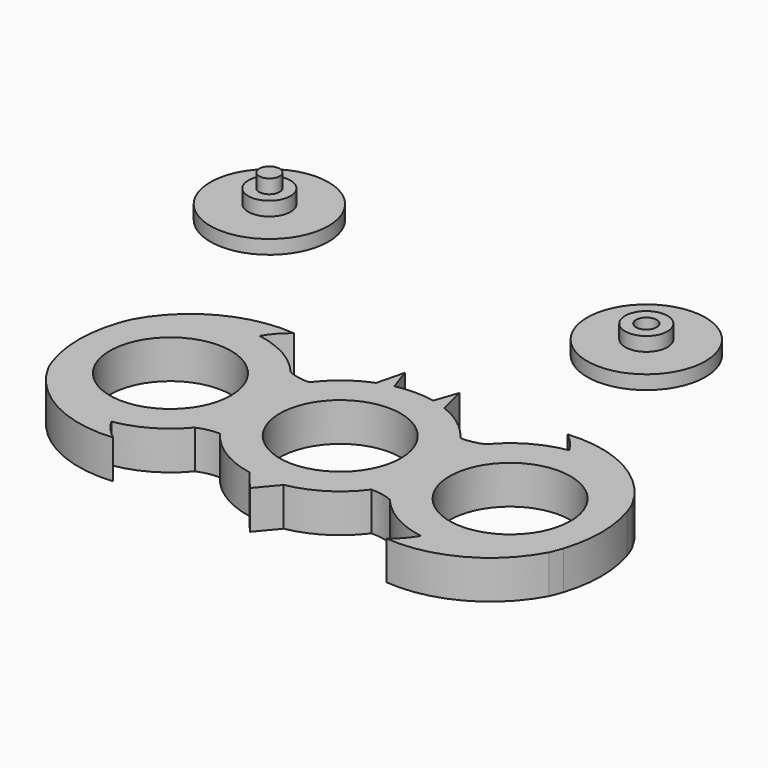
from build123d import *

# Parameters (mm, degrees)
F0_R     = 11.055
F1_DEPTH = 7.04
F2_R     = 3.8608
F2_R_2   = 1.8669
F3_DEPTH = 5.08
F2_R_3   = 10.795
F4_DEPTH = 2.54
F5_DEPTH = 7.62


with BuildPart() as f1:
    # F0 (on Top) → F1 (new body)
    with BuildSketch(Plane.XY):
        with BuildLine():
            ThreePointArc((-46.5429451347, 7.2365655902), (-39.0213444379, 15.1528564439), (-28.2458606842, 16.9223444484))
            ThreePointArc((-28.2458606842, 16.9223444484), (-26.7954522093, 18.9396770038), (-24.9616837395, 20.6161639804))
            ThreePointArc((-24.9616837395, 20.6161639804), (-37.0112899435, 18.1759091976), (-45.6916782608, 9.4696636386))
            ThreePointArc((-45.6916782608, 9.4696636386), (-46.1457401666, 8.3639516727), (-46.5429451347, 7.2365655902))
        make_face()
        with BuildLine():
            ThreePointArc((-28.2458606842, -16.9223444484), (-39.0213444379, -15.1528564439), (-46.5429451347, -7.2365655902))
            ThreePointArc((-46.5429451347, -7.2365655902), (-46.1457401666, -8.3639516727), (-45.6916782608, -9.4696636386))
            ThreePointArc((-45.6916782608, -9.4696636386), (-37.0112899435, -18.1759091976), (-24.9616837395, -20.6161639804))
            ThreePointArc((-24.9616837395, -20.6161639804), (-26.7954522093, -18.9396770038), (-28.2458606842, -16.9223444484))
        make_face()
        with BuildLine():
            ThreePointArc((-13.8011629931, 10.1724591441), (-15.8450830005, 10.3315929693), (-17.8017727644, 10.9433917429))
            ThreePointArc((-17.8017727644, 10.9433917429), (-16.5374743475, 9.2079518218), (-15.5, 7.3280983208))
            ThreePointArc((-15.5, 7.3280983208), (-14.7194475205, 8.7914099944), (-13.8011629931, 10.1724591441))
        make_face()
        with BuildLine():
            ThreePointArc((-13.855, 0), (-14.27130422, 3.7552313511), (-15.5, 7.3280983208))
            ThreePointArc((-15.5, 7.3280983208), (-17.145, 0), (-15.5, -7.3280983208))
            ThreePointArc((-15.5, -7.3280983208), (-14.27130422, -3.7552313511), (-13.855, 0))
        make_face()
        with BuildLine():
            ThreePointArc((-13.8011629931, -10.1724591441), (-14.7194475205, -8.7914099944), (-15.5, -7.3280983208))
            ThreePointArc((-15.5, -7.3280983208), (-16.5374743475, -9.2079518218), (-17.8017727644, -10.9433917429))
            ThreePointArc((-17.8017727644, -10.9433917429), (-15.8450830005, -10.3315929693), (-13.8011629931, -10.1724591441))
        make_face()
        with BuildLine():
            ThreePointArc((-13.8011629931, 10.1724591441), (-14.7194475205, 8.7914099944), (-15.5, 7.3280983208))
            ThreePointArc((-15.5, 7.3280983208), (-14.27130422, 3.7552313511), (-13.855, 0))
            ThreePointArc((-13.855, 0), (-14.27130422, -3.7552313511), (-15.5, -7.3280983208))
            ThreePointArc((-15.5, -7.3280983208), (-14.7194475205, -8.7914099944), (-13.8011629931, -10.1724591441))
            ThreePointArc((-13.8011629931, -10.1724591441), (-9.0876766021, -14.5384029032), (-3.0980425219, -16.862774313))
            ThreePointArc((-3.0980425219, -16.862774313), (0.0279613173, -17.1449771993), (3.1530280548, -16.8525795974))
            ThreePointArc((3.1530280548, -16.8525795974), (9.1113748051, -14.5235627227), (13.8011629931, -10.1724591441))
            ThreePointArc((13.8011629931, -10.1724591441), (14.7194475205, -8.7914099944), (15.5, -7.3280983208))
            ThreePointArc((15.5, -7.3280983208), (13.855, 0), (15.5, 7.3280983208))
            ThreePointArc((15.5, 7.3280983208), (14.7194475205, 8.7914099944), (13.8011629931, 10.1724591441))
            ThreePointArc((13.8011629931, 10.1724591441), (10.4277783329, 13.609278601), (6.2316875055, 15.9723854146))
            ThreePointArc((6.2316875055, 15.9723854146), (4.9049913789, 16.4283926351), (3.5454552824, 16.7744082411))
            ThreePointArc((3.5454552824, 16.7744082411), (0, 17.145), (-3.5454552824, 16.7744082411))
            ThreePointArc((-3.5454552824, 16.7744082411), (-4.9049913789, 16.4283926351), (-6.2316875055, 15.9723854146))
            ThreePointArc((-6.2316875055, 15.9723854146), (-10.4277783329, 13.609278601), (-13.8011629931, 10.1724591441))
        make_face()
        Circle(F0_R, mode=Mode.SUBTRACT)
        with BuildLine():
            Line((-4.9772132188, 20.9476407617), (-6.2316875055, 15.9723854146))
            ThreePointArc((-6.2316875055, 15.9723854146), (-4.9049913789, 16.4283926351), (-3.5454552824, 16.7744082411))
            Line((-3.5454552824, 16.7744082411), (-4.9772132188, 20.9476407617))
        make_face()
        with BuildLine():
            Line((4.9772132188, 20.9476407617), (3.5454552824, 16.7744082411))
            ThreePointArc((3.5454552824, 16.7744082411), (4.9049913789, 16.4283926351), (6.2316875055, 15.9723854146))
            Line((6.2316875055, 15.9723854146), (4.9772132188, 20.9476407617))
        make_face()
        with BuildLine():
            ThreePointArc((3.1530280548, -16.8525795974), (0.0279613173, -17.1449771993), (-3.0980425219, -16.862774313))
            Line((-3.0980425219, -16.862774313), (0, -20.6161639804))
            Line((0, -20.6161639804), (3.1530280548, -16.8525795974))
        make_face()
        with BuildLine():
            ThreePointArc((15.5, 7.3280983208), (13.855, 0), (15.5, -7.3280983208))
            ThreePointArc((15.5, -7.3280983208), (16.72869578, -3.7552313511), (17.145, 0))
            ThreePointArc((17.145, 0), (16.72869578, 3.7552313511), (15.5, 7.3280983208))
        make_face()
        with BuildLine():
            ThreePointArc((17.8017727644, 10.9433917429), (15.8450830005, 10.3315929693), (13.8011629931, 10.1724591441))
            ThreePointArc((13.8011629931, 10.1724591441), (14.7194475205, 8.7914099944), (15.5, 7.3280983208))
            ThreePointArc((15.5, 7.3280983208), (16.5374743475, 9.2079518218), (17.8017727644, 10.9433917429))
        make_face()
        with BuildLine():
            ThreePointArc((15.5, -7.3280983208), (14.7194475205, -8.7914099944), (13.8011629931, -10.1724591441))
            ThreePointArc((13.8011629931, -10.1724591441), (15.8450830005, -10.3315929693), (17.8017727644, -10.9433917429))
            ThreePointArc((17.8017727644, -10.9433917429), (16.5374743475, -9.2079518218), (15.5, -7.3280983208))
        make_face()
        with BuildLine():
            ThreePointArc((17.145, 0), (16.72869578, -3.7552313511), (15.5, -7.3280983208))
            ThreePointArc((15.5, -7.3280983208), (16.5374743475, -9.2079518218), (17.8017727644, -10.9433917429))
            ThreePointArc((17.8017727644, -10.9433917429), (22.4819915173, -14.8793332004), (28.2458606842, -16.9223444484))
            ThreePointArc((28.2458606842, -16.9223444484), (39.0213444379, -15.1528564439), (46.5429451347, -7.2365655902))
            ThreePointArc((46.5429451347, -7.2365655902), (47.6858732568, 0), (46.5429451347, 7.2365655902))
            ThreePointArc((46.5429451347, 7.2365655902), (39.0213444379, 15.1528564439), (28.2458606842, 16.9223444484))
            ThreePointArc((28.2458606842, 16.9223444484), (22.4819915173, 14.8793332004), (17.8017727644, 10.9433917429))
            ThreePointArc((17.8017727644, 10.9433917429), (16.5374743475, 9.2079518218), (15.5, 7.3280983208))
            ThreePointArc((15.5, 7.3280983208), (16.72869578, 3.7552313511), (17.145, 0))
        make_face()
        with Locations((31, 0)):
            Circle(F0_R, mode=Mode.SUBTRACT)
        with BuildLine():
            ThreePointArc((24.9616837395, 20.6161639804), (26.7954522093, 18.9396770038), (28.2458606842, 16.9223444484))
            ThreePointArc((28.2458606842, 16.9223444484), (39.0213444379, 15.1528564439), (46.5429451347, 7.2365655902))
            ThreePointArc((46.5429451347, 7.2365655902), (46.1457401666, 8.3639516727), (45.6916782608, 9.4696636386))
            ThreePointArc((45.6916782608, 9.4696636386), (37.0112899435, 18.1759091976), (24.9616837395, 20.6161639804))
        make_face()
        with BuildLine():
            ThreePointArc((46.5429451347, -7.2365655902), (39.0213444379, -15.1528564439), (28.2458606842, -16.9223444484))
            ThreePointArc((28.2458606842, -16.9223444484), (26.7954522093, -18.9396770038), (24.9616837395, -20.6161639804))
            ThreePointArc((24.9616837395, -20.6161639804), (37.0112899435, -18.1759091976), (45.6916782608, -9.4696636386))
            ThreePointArc((45.6916782608, -9.4696636386), (46.1457401666, -8.3639516727), (46.5429451347, -7.2365655902))
        make_face()
        with BuildLine():
            ThreePointArc((-15.5, 7.3280983208), (-16.5374743475, 9.2079518218), (-17.8017727644, 10.9433917429))
            ThreePointArc((-17.8017727644, 10.9433917429), (-22.4819915173, 14.8793332004), (-28.2458606842, 16.9223444484))
            ThreePointArc((-28.2458606842, 16.9223444484), (-39.0213444379, 15.1528564439), (-46.5429451347, 7.2365655902))
            ThreePointArc((-46.5429451347, 7.2365655902), (-47.6858732568, 0), (-46.5429451347, -7.2365655902))
            ThreePointArc((-46.5429451347, -7.2365655902), (-39.0213444379, -15.1528564439), (-28.2458606842, -16.9223444484))
            ThreePointArc((-28.2458606842, -16.9223444484), (-22.4819915173, -14.8793332004), (-17.8017727644, -10.9433917429))
            ThreePointArc((-17.8017727644, -10.9433917429), (-16.5374743475, -9.2079518218), (-15.5, -7.3280983208))
            ThreePointArc((-15.5, -7.3280983208), (-17.145, 0), (-15.5, 7.3280983208))
        make_face()
        with Locations((-31, 0)):
            Circle(F0_R, mode=Mode.SUBTRACT)
    extrude(amount=F1_DEPTH)


with BuildPart() as f3:
    # F2 (on Top) → F3 (new body)
    with BuildSketch(Plane.XY):
        with Locations((-57.9895079136, 56.3239566982)):
            Circle(F2_R)
        with Locations((-57.9895079136, 56.3239566982)):
            Circle(F2_R_2, mode=Mode.SUBTRACT)
    extrude(amount=F3_DEPTH)

    # F2 (on Top) → F4 (join)
    with BuildSketch(Plane.XY):
        with Locations((-57.9895079136, 56.3239566982)):
            Circle(F2_R_3)
        with Locations((-57.9895079136, 56.3239566982)):
            Circle(F2_R, mode=Mode.SUBTRACT)
    extrude(amount=F4_DEPTH)

    # F2 (on Top) → F5 (join)
    with BuildSketch(Plane.XY):
        with Locations((-57.9895079136, 56.3239566982)):
            Circle(F2_R_2)
    extrude(amount=F5_DEPTH)


with BuildPart() as f3b:
    # F2 (on Top) → F3, piece 2 (new body)
    with BuildSketch(Plane.XY):
        with Locations((10.053133592, 57.2697557509)):
            Circle(F2_R)
        with Locations((10.053133592, 57.2697557509)):
            Circle(F2_R_2, mode=Mode.SUBTRACT)
    extrude(amount=F3_DEPTH)


with BuildPart() as f4:
    # F2 (on Top) → F4, piece 2 (new body)
    with BuildSketch(Plane.XY):
        with Locations((10.053133592, 57.2697557509)):
            Circle(F2_R_3)
        with Locations((10.053133592, 57.2697557509)):
            Circle(F2_R, mode=Mode.SUBTRACT)
    extrude(amount=F4_DEPTH)


solid = Compound([f1.part, f3.part, f3b.part, f4.part])
